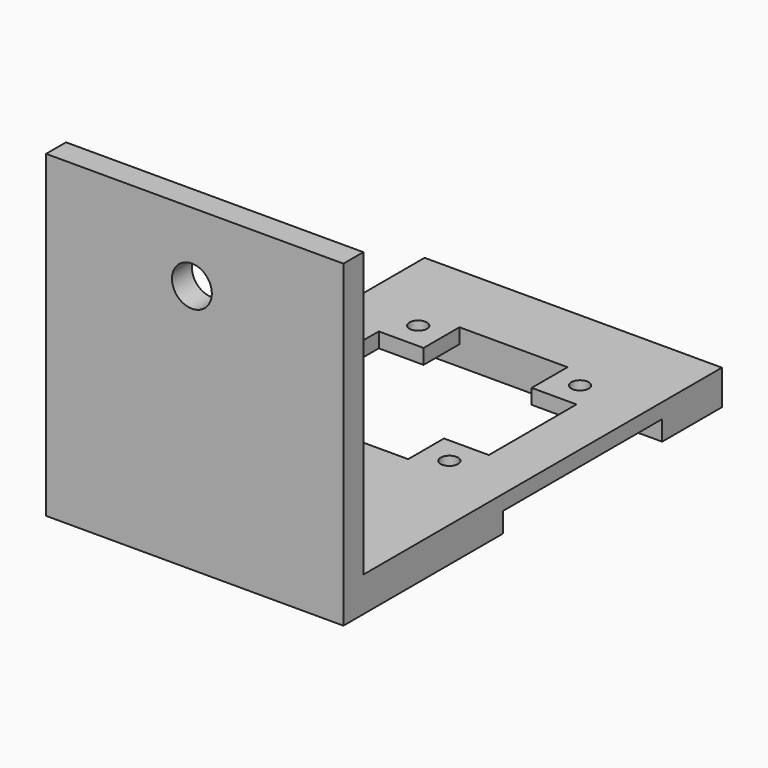
from build123d import *

# Parameters (mm, degrees)
F0_W     = 10
F0_H     = 10
F0_W_2   = 9
F0_H_2   = 9
F0_R     = 1.75
F0_R_2   = 1.9678984668
F1_DEPTH = 3
F0_W_3   = 59.7
F0_H_3   = 5
F2_DEPTH = 60
F4_D     = 8
F6_DEPTH = 4
F8_D     = 8


# Not quite as in the source:
# - a feature names something its author has since deleted; it is built from what else it names


with BuildPart() as f1:
    # F0 (on Top) → F1 (new body)
    with BuildSketch(Plane.XY):
        with Locations((9.4588409364, 5)):
            Rectangle(F0_W, F0_H)
        with Locations((59.1588409364, 5)):
            Rectangle(F0_W, F0_H)
        Polygon((14.4588409364, 10), (14.4588409364, 0), (23.4588409364, 0), (45.1588409364, 0), (54.1588409364, 0), (54.1588409364, 10), align=None)
        Polygon((14.4588409364, -9), (14.4588409364, 0), (4.4588409364, 0), (4.4588409364, -40), (14.4588409364, -40), (14.4588409364, -31), align=None)
        Polygon((64.1588409364, 0), (54.1588409364, 0), (54.1588409364, -9), (54.1588409364, -31), (54.1588409364, -40), (64.1588409364, -40), align=None)
        Polygon((14.4588409364, -40), (4.4588409364, -40), (4.4588409364, -50), (4.4588409364, -75), (64.1588409364, -75), (64.1588409364, -50), (64.1588409364, -40), (54.1588409364, -40), (45.1588409364, -40), (23.4588409364, -40), align=None)
        with Locations((18.9588409364, -4.5)):
            Rectangle(F0_W_2, F0_H_2)
        with Locations((18.0588409364, -3.6)):
            Circle(F0_R, mode=Mode.SUBTRACT)
        with Locations((49.6588409364, -4.5)):
            Rectangle(F0_W_2, F0_H_2)
        with Locations((50.5588409364, -3.6)):
            Circle(F0_R, mode=Mode.SUBTRACT)
        with Locations((18.9588409364, -35.5)):
            Rectangle(F0_W_2, F0_H_2)
        with Locations((18.2767394032, -36.1821015332)):
            Circle(F0_R_2, mode=Mode.SUBTRACT)
        with Locations((49.6588409364, -35.5)):
            Rectangle(F0_W_2, F0_H_2)
        with Locations((50.5588409364, -36.4)):
            Circle(F0_R, mode=Mode.SUBTRACT)
        Polygon((4.4588409364, 10), (14.4588409364, 10), (54.1588409364, 10), (64.1588409364, 10), (64.1588409364, 15), (4.4588409364, 15), align=None)
    extrude(amount=F1_DEPTH)

    # F0 (on Top) → F2 (join)
    with BuildSketch(Plane.XY):
        with Locations((34.3088409364, -77.5)):
            Rectangle(F0_W_3, F0_H_3)
    extrude(amount=F2_DEPTH)

    # F4 (through all)
    with Locations(Plane.XZ.offset(80)):
        with Locations((33.7338409364, 46.1369195342)):
            Hole(F4_D / 2)

    # F5 (on face) → F6 (join)
    with BuildSketch(Plane(origin=(0, 0, 0), x_dir=(1, 0, 0), z_dir=(0, 0, -1))):
        Polygon((4.4588409364, 40), (23.4588409364, 40), (45.1588409364, 40), (64.1588409364, 40), (64.1588409364, 80), (4.4588409364, 80), align=None)
        Polygon((23.4588409364, 0), (4.4588409364, 0), (4.4588409364, -10), (4.4588409364, -15), (64.1588409364, -15), (64.1588409364, -10), (64.1588409364, 0), (45.1588409364, 0), align=None)
    extrude(amount=F6_DEPTH)

    # F8 (through all)
    with Locations(Plane.XY.offset(3)):
        with Locations((34.1588409364, -55.4992741766)):
            Hole(F8_D / 2)


solid = f1.part
